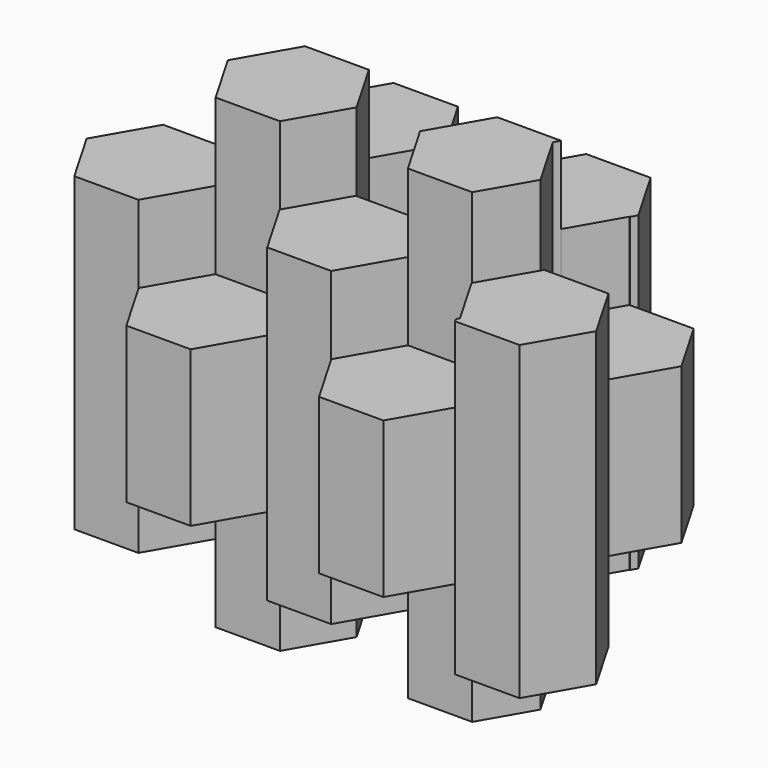
from build123d import *

# Parameters (mm, degrees)
F1_DEPTH      = 25.4
F1_DEPTH_BACK = 25.4
F2_DEPTH      = 50.8
F2_DEPTH_BACK = 50.8
F3_DEPTH      = 76.2
F3_DEPTH_BACK = 76.2


# Not quite as in the source:
# - ends of sketch curves that miss each other by under 0.0002 mm in the source are joined


with BuildPart() as f1:
    # F0 (on Top) → F1 (new body, two sides)
    with BuildSketch(Plane.XY) as f1_sk:
        Polygon((-34.353646, 7.18203), (-23.898079, 25.341705), (-23.965786, 25.458653), (-34.421353, 7.298978), align=None)
        Polygon((-55.38092, 7.11486), (-34.412292, 7.139928), (-34.421353, 7.155578), (-55.389981, 7.130511), align=None)
        Polygon((-34.377863, 7.139969), (-34.353646, 7.18203), (-34.421353, 7.298978), (-23.965786, 25.458653), (-34.421353, 43.518332), (-55.42441, 43.493223), (-65.904194, 25.291487), (-55.389981, 7.130511), (-34.421353, 7.155578), (-34.412292, 7.139928), align=None)
    extrude(amount=F1_DEPTH)
    extrude(f1_sk.sketch, amount=-F1_DEPTH_BACK)


with BuildPart() as f1b:
    # F0 (on Top) → F1, piece 2 (new body, two sides)
    with BuildSketch(Plane.XY) as f1_2_sk:
        Polygon((-23.898079, -11.021049), (-23.935389, -10.956603), (-23.941568, -10.95661), (-34.421352, -29.158346), (-34.384041, -29.222792), (-34.377863, -29.222784), align=None)
        Polygon((7.584763, -29.108128), (-2.938511, -10.931502), (-3.004525, -11.046158), (7.518749, -29.222785), align=None)
        Polygon((-2.938511, -10.931502), (-23.935389, -10.956603), (-23.898079, -11.021049), (-34.377863, -29.222784), (-34.384041, -29.222792), (-23.898078, -47.334973), (-2.895021, -47.309864), (7.518749, -29.222785), (-3.004525, -11.046158), align=None)
    extrude(amount=F1_DEPTH)
    extrude(f1_2_sk.sketch, amount=-F1_DEPTH_BACK)


with BuildPart() as f1c:
    # F0 (on Top) → F1, piece 3 (new body, two sides)
    with BuildSketch(Plane.XY) as f1_3_sk:
        Polygon((7.541273, 43.727559), (-2.938511, 25.525823), (-2.895021, 25.525875), (7.584763, 43.72761), align=None)
        Polygon((39.067603, 25.576041), (28.54433, 43.752668), (28.523653, 43.716755), (39.046927, 25.540128), align=None)
        Polygon((-2.938511, 25.525823), (7.584762, 7.349196), (28.424096, 7.374109), (38.875079, 25.525822), (39.038803, 25.526018), (39.046927, 25.540128), (28.523653, 43.716755), (28.54433, 43.752668), (7.584763, 43.727611), (-2.895021, 25.525875), align=None)
    extrude(amount=F1_DEPTH)
    extrude(f1_3_sk.sketch, amount=-F1_DEPTH_BACK)


with BuildPart() as f1d:
    # F0 (on Top) → F1, piece 4 (new body, two sides)
    with BuildSketch(Plane.XY) as f1_4_sk:
        Polygon((69.211585, 41.761663), (59.886261, 25.565041), (60.049984, 25.565237), (69.375308, 41.761859), align=None)
        Polygon((59.886261, 25.565041), (59.878137, 25.550931), (70.40141, 7.374305), (69.255075, 5.383301), (90.258132, 5.408409), (100.737916, 23.610145), (90.214642, 41.786772), (69.375308, 41.761859), (60.049984, 25.565237), align=None)
    extrude(amount=F1_DEPTH)
    extrude(f1_4_sk.sketch, amount=-F1_DEPTH_BACK)


with BuildPart() as f1e:
    # F0 (on Top) → F1, piece 5 (new body, two sides)
    with BuildSketch(Plane.XY) as f1_5_sk:
        Polygon((70.001467, -30.065401), (70.550445, -29.111913), (60.660062, -12.028465), (60.111084, -12.981953), align=None)
        Polygon((60.070661, -47.313649), (70.001467, -30.065401), (60.111084, -12.981953), (60.660062, -12.028465), (60.027171, -10.935286), (39.024114, -10.960395), (28.54433, -29.162131), (39.067604, -47.338758), align=None)
    extrude(amount=F1_DEPTH)
    extrude(f1_5_sk.sketch, amount=-F1_DEPTH_BACK)


with BuildPart() as f2:
    # F0 (on Top) → F2 (new body, two sides)
    with BuildSketch(Plane.XY) as f2_sk:
        Polygon((-23.935389, -10.956603), (-34.412292, 7.139928), (-55.38092, 7.11486), (-55.389981, 7.130511), (-55.42441, 7.130469), (-65.904194, -11.071266), (-55.38092, -29.247893), (-34.384041, -29.222792), (-34.421352, -29.158346), (-23.941568, -10.95661), align=None)
    extrude(amount=F2_DEPTH)
    extrude(f2_sk.sketch, amount=-F2_DEPTH_BACK)


with BuildPart() as f2b:
    # F0 (on Top) → F2, piece 2 (new body, two sides)
    with BuildSketch(Plane.XY) as f2_2_sk:
        Polygon((7.475259, 7.155578), (-2.938511, -10.931502), (7.584763, -29.108128), (7.518749, -29.222785), (28.521806, -29.197676), (39.00159, -10.99594), (38.918569, -10.85254), (28.478316, 7.180687), align=None)
    extrude(amount=F2_DEPTH)
    extrude(f2_2_sk.sketch, amount=-F2_DEPTH_BACK)


with BuildPart() as f2c:
    # F0 (on Top) → F2, piece 3 (new body, two sides)
    with BuildSketch(Plane.XY) as f2_3_sk:
        Polygon((60.660062, -12.028465), (70.550445, -29.111913), (70.001467, -30.065401), (70.634358, -31.15858), (91.637415, -31.133471), (102.117199, -12.931735), (91.593925, 5.244892), (70.590868, 5.219783), align=None)
    extrude(amount=F2_DEPTH)
    extrude(f2_3_sk.sketch, amount=-F2_DEPTH_BACK)


with BuildPart() as f2d:
    # F0 (on Top) → F2, piece 4 (new body, two sides)
    with BuildSketch(Plane.XY) as f2_4_sk:
        Polygon((39.003437, 61.918491), (28.54433, 43.752668), (39.067603, 25.576041), (39.046927, 25.540128), (59.886261, 25.565041), (69.211585, 41.761663), (69.375308, 41.761859), (70.529768, 43.766973), (60.006494, 61.9436), align=None)
    extrude(amount=F2_DEPTH)
    extrude(f2_4_sk.sketch, amount=-F2_DEPTH_BACK)


with BuildPart() as f2e:
    # F0 (on Top) → F2, piece 5 (new body, two sides)
    with BuildSketch(Plane.XY) as f2_5_sk:
        Polygon((-34.421352, 43.677393), (-23.898078, 25.500766), (-2.938511, 25.525823), (7.541273, 43.727559), (7.584763, 43.727611), (-2.938511, 61.904237), (-23.941568, 61.879128), align=None)
    extrude(amount=F2_DEPTH)
    extrude(f2_5_sk.sketch, amount=-F2_DEPTH_BACK)


with BuildPart() as f3:
    # F0 (on Top) → F3 (new body, two sides)
    with BuildSketch(Plane.XY) as f3_sk:
        Polygon((-23.965786, 25.458653), (-23.898079, 25.341705), (-34.353646, 7.18203), (-23.898079, -10.877648), (-2.895022, -10.85254), (7.584762, 7.349196), (-2.938511, 25.525823), (-23.898078, 25.500766), (-23.941569, 25.500714), align=None)
    extrude(amount=F3_DEPTH)
    extrude(f3_sk.sketch, amount=-F3_DEPTH_BACK)


with BuildPart() as f3b:
    # F0 (on Top) → F3, piece 2 (new body, two sides)
    with BuildSketch(Plane.XY) as f3_2_sk:
        Polygon((28.58782, 7.374305), (28.424096, 7.374109), (28.395295, 7.324087), (28.478316, 7.180687), (38.918569, -10.85254), (59.921626, -10.827431), (69.255075, 5.383301), (58.731801, 23.559927), (59.878137, 25.550931), (39.038803, 25.526018), align=None)
    extrude(amount=F3_DEPTH)
    extrude(f3_2_sk.sketch, amount=-F3_DEPTH_BACK)


solid = Compound([f1.part, f1b.part, f1c.part, f1d.part, f1e.part, f2.part, f2b.part, f2c.part, f2d.part, f2e.part, f3.part, f3b.part])
